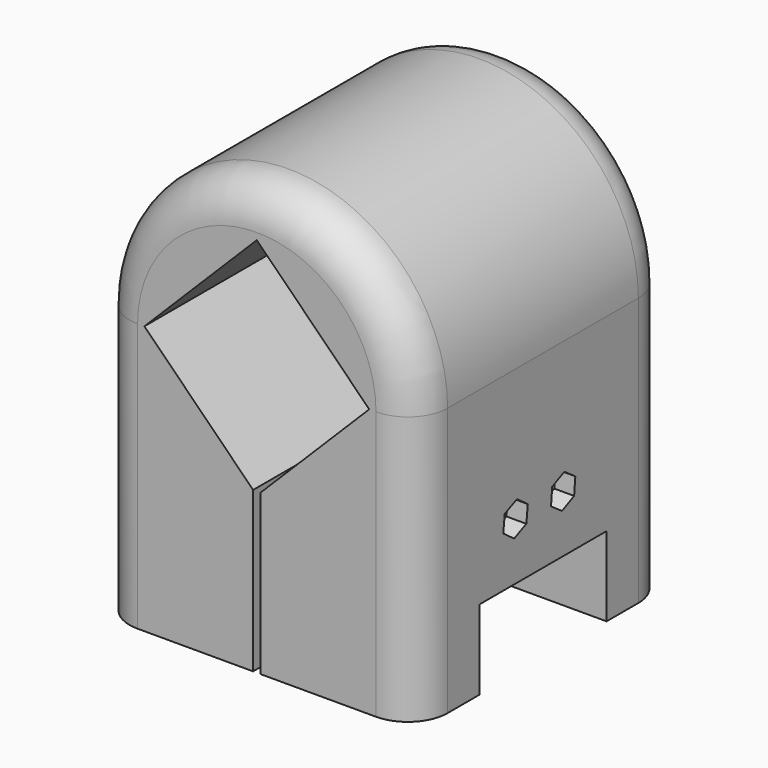
from build123d import *

# Parameters (mm, degrees)
F3_DEPTH = 101.6
F4_DEPTH = 282.663077116
F5_R     = 3.175
F6_DEPTH = 127
F7_DEPTH = 6.35
F8_W     = 50.8
F8_H     = 50.8
F8_H_2   = 25.4
F9_DEPTH = 127
F10_R    = 12.7


with BuildPart() as f3:
    # F0 (on Front) → F3 (new body)
    with BuildSketch(Plane.XZ):
        with BuildLine():
            Line((50.8, -85.7884685198), (50.8, 0))
            ThreePointArc((50.8, 0), (0, -50.8), (-50.8, 0))
            Line((-50.8, 0), (-50.8, -85.7884685198))
            Line((-50.8, -85.7884685198), (50.8, -85.7884685198))
        make_face()
        with BuildLine():
            ThreePointArc((-50.8, 0), (0, -50.8), (50.8, 0))
            ThreePointArc((50.8, 0), (0, 50.8), (-50.8, 0))
        make_face()
    extrude(amount=F3_DEPTH)

    # F2 (on face) + F1 (on Front) → F4 (cut)
    with BuildSketch(Plane.XZ):
        with BuildLine():
            Line((-1.1809319258, -85.7884685198), (1.1809319258, -85.7884685198))
            Line((1.1809319258, -85.7884685198), (1.1809319258, -50.786271765))
            ThreePointArc((1.1809319258, -50.786271765), (0, -50.8), (-1.1809319258, -50.786271765))
            Line((-1.1809319258, -50.786271765), (-1.1809319258, -85.7884685198))
        make_face()
        with BuildLine():
            ThreePointArc((-1.1809319258, -50.786271765), (0, -50.8), (1.1809319258, -50.786271765))
            Line((1.1809319258, -50.786271765), (1.1809319258, 14.9626284838))
            Line((1.1809319258, 14.9626284838), (-1.1809319258, 14.9626284838))
            Line((-1.1809319258, 14.9626284838), (-1.1809319258, -50.786271765))
        make_face()
    with BuildSketch(Plane.XZ):
        Polygon((35.9210244843, 0), (0, 35.9210244843), (-35.9210244843, 0), (0, -35.9210244843), align=None)
    extrude(amount=F4_DEPTH, mode=Mode.SUBTRACT)

    # F5 (on face) → F6 (cut)
    with BuildSketch(Plane.YZ.offset(50.8)):
        with Locations((-42.7350864422, -42.1568825841)):
            Circle(F5_R)
        with Locations((-61.7602499746, -42.1568825841)):
            Circle(F5_R)
    extrude(amount=-F6_DEPTH, mode=Mode.SUBTRACT)

    # F5 (on face) → F7 (cut)
    with BuildSketch(Plane.YZ.offset(50.8)):
        Polygon((-62.336745475, -47.4765820931), (-57.4415028095, -45.3159920871), (-56.8650073091, -39.9962925781), (-61.1837544742, -36.8371830751), (-66.0789971397, -38.9977730811), (-66.6554926401, -44.3174725901), align=None)
        with Locations((-61.7602499746, -42.1568825841)):
            Circle(F5_R, mode=Mode.SUBTRACT)
        Polygon((-43.2069172048, -47.486893887), (-38.3550766327, -45.2305056623), (-37.88324587, -39.9004943594), (-42.2632556795, -36.8268712812), (-47.1150962516, -39.0832595059), (-47.5869270143, -44.4132708088), align=None)
        with Locations((-42.7350864422, -42.1568825841)):
            Circle(F5_R, mode=Mode.SUBTRACT)
    extrude(amount=-F7_DEPTH, mode=Mode.SUBTRACT)

    # F8 (on face) → F9 (cut)
    with BuildSketch(Plane.YZ.offset(50.8)):
        with Locations((-50.8, -85.7884685198)):
            Rectangle(F8_W, F8_H)
        with Locations((-50.8, -73.0884685198)):
            Rectangle(F8_W, F8_H_2)
    extrude(amount=-F9_DEPTH, mode=Mode.SUBTRACT)

    # F10
    f10_edges = [f3.edges().sort_by_distance(p)[0] for p in [
        (0, -101.6, 50.8),
        (50.8, -101.6, -42.894234),
        (0, 0, 50.8),
        (50.8, 0, -42.894234),
        (-50.8, 0, -42.894234),
        (-50.8, -101.6, -42.894234),
    ]]
    fillet(f10_edges, radius=F10_R)


solid = f3.part
